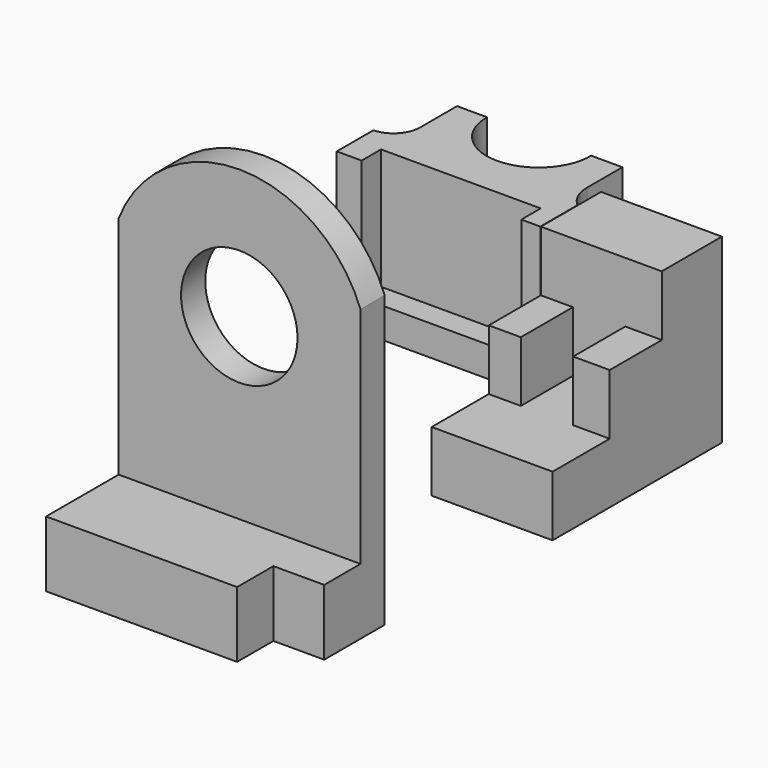
from build123d import *
from build123d import SkipClean  # not in build123d's __all__

# Parameters (mm, degrees)
F0_W      = 25.4
F0_H      = 44.45
F1_DEPTH  = 12.7
F2_W      = 25.4
F2_H      = 29.4602914497
F3_DEPTH  = 12.7
F4_W      = 10.9979929402
F4_H      = 13.6651070789
F5_DEPTH  = 12.7
F7_DEPTH  = 12.7
F8_W      = 50.8
F8_H      = 25.4
F9_DEPTH  = 101.6
F11_DEPTH = 25.4
F12_R     = 12.2295787835
F13_DEPTH = 25.4
F14_R     = 12.2295787835
F15_DEPTH = 19.05
F16_W     = 10.6714690655
F16_H     = 9.525
F17_DEPTH = 25.4
F19_DEPTH = 6.35
F21_DEPTH = 25.4
F23_DEPTH = 25.4


with BuildPart() as f1:
    # F0 (on Top) → F1 (new body)
    with BuildSketch(Plane.XY):
        with Locations((12.7, 22.225)):
            Rectangle(F0_W, F0_H)
    extrude(amount=F1_DEPTH)

    # F2 (on face) → F3 (join)
    with BuildSketch(Plane.XY.offset(12.7)):
        with Locations((12.7, 29.7198542751)):
            Rectangle(F2_W, F2_H)
    extrude(amount=F3_DEPTH)

    # F4 (on face) → F5 (cut)
    with BuildSketch(Plane.XY.offset(25.4)):
        with Locations((12.2352666222, 21.8222620897)):
            Rectangle(F4_W, F4_H)
    extrude(amount=-F5_DEPTH, mode=Mode.SUBTRACT)

    # F6 (on face) → F7 (join)
    with BuildSketch(Plane.XY.offset(25.4)):
        Polygon((25.4, 44.45), (0, 44.45), (0, 28.6548156291), (6.736270152, 28.6548156291), (17.7342630923, 28.6548156291), (25.4, 28.6548156291), align=None)
    extrude(amount=F7_DEPTH)

    # F18 (on Top) → F19 (join)
    with BuildSketch(Plane.XY):
        with BuildLine():
            Line((-3.81, 63.023544848), (-53.6545139277, 63.023544848))
            ThreePointArc((-53.6545139277, 63.023544848), (-56.348590764, 61.9076216843), (-57.4645139277, 59.213544848))
            Line((-57.4645139277, 59.213544848), (-57.4645139277, 38.1405837834))
            Line((-57.4645139277, 38.1405837834), (0, 38.1405837834))
            Line((0, 38.1405837834), (0, 59.213544848))
            ThreePointArc((0, 59.213544848), (-1.1159231637, 61.9076216843), (-3.81, 63.023544848))
        make_face()
    extrude(amount=F19_DEPTH)

    # F20 (on face) → F21 (cut)
    with BuildSketch(Plane.XY.offset(6.35)):
        with BuildLine():
            Line((-16.9094149023, 63.023544848), (-38.7679263949, 63.023544848))
            ThreePointArc((-38.7679263949, 63.023544848), (-27.8386706486, 51.9472434828), (-16.9094149023, 63.023544848))
        make_face()
    extrude(amount=-F21_DEPTH, mode=Mode.SUBTRACT)

    # F22 (on face) → F23 (join)
    with BuildSketch(Plane.XY.offset(6.35)):
        with BuildLine():
            Line((-45.2292449772, 38.1405837834), (-45.2292449772, 43.2271584868))
            Line((-45.2292449772, 43.2271584868), (-11.6853676736, 43.2271584868))
            Line((-11.6853676736, 43.2271584868), (-11.6853676736, 38.1405837834))
            Line((-11.6853676736, 38.1405837834), (-7.6985950582, 38.1405837834))
            Line((-7.6985950582, 38.1405837834), (-7.6985950582, 47.9013063014))
            ThreePointArc((-7.6985950582, 47.9013063014), (-9.6624188313, 50.4964154712), (-10.3597074512, 53.6752492189))
            Line((-10.3597074512, 53.6752492189), (-10.3597074512, 63.023544848))
            Line((-10.3597074512, 63.023544848), (-16.9094149023, 63.023544848))
            ThreePointArc((-16.9094149023, 63.023544848), (-27.8386706486, 51.9472434828), (-38.7679263949, 63.023544848))
            Line((-38.7679263949, 63.023544848), (-45.0917705894, 63.023544848))
            Line((-45.0917705894, 63.023544848), (-45.0917705894, 53.2628260553))
            ThreePointArc((-45.0917705894, 53.2628260553), (-46.6539859613, 49.4227442996), (-50.4532940686, 47.7638281882))
            Line((-50.4532940686, 47.7638281882), (-50.4532940686, 38.1405837834))
            Line((-50.4532940686, 38.1405837834), (-45.2292449772, 38.1405837834))
        make_face()
    with SkipClean():  # cleaning this boolean's faces spoils the solid; the shape is the same uncleaned
        extrude(amount=F23_DEPTH)


with BuildPart() as f9:
    # F8 (on Top) → F9 (new body)
    with BuildSketch(Plane.XY):
        with Locations((-2.7682126224, -53.3297498107)):
            Rectangle(F8_W, F8_H)
    extrude(amount=F9_DEPTH)

    # F10 (on face) → F11 (cut)
    with BuildSketch(Plane.XZ.offset(66.0297498107)):
        with BuildLine():
            ThreePointArc((-28.1682126224, 61.2272843719), (-2.6642465557, 78.5167686352), (22.6317873776, 60.9244629741))
            Line((22.6317873776, 60.9244629741), (22.6317873776, 101.6))
            Line((22.6317873776, 101.6), (-28.1682126224, 101.6))
            Line((-28.1682126224, 101.6), (-28.1682126224, 61.2272843719))
        make_face()
    extrude(amount=-F11_DEPTH, mode=Mode.SUBTRACT)

    # F12 (on face) → F13 (cut)
    with BuildSketch(Plane.XZ.offset(66.0297498107)):
        with Locations((-2.826482869, 51.3007106537)):
            Circle(F12_R)
    extrude(amount=-F13_DEPTH, mode=Mode.SUBTRACT)

    # F14 (on face) → F15 (cut)
    with BuildSketch(Plane.XZ.offset(66.0297498107)):
        with BuildLine():
            Line((-28.1682126224, 61.2272843719), (-28.1682126224, 13.8355828822))
            Line((-28.1682126224, 13.8355828822), (22.6317873776, 13.8355828822))
            Line((22.6317873776, 13.8355828822), (22.6317873776, 60.9244629741))
            ThreePointArc((22.6317873776, 60.9244629741), (-2.6642465557, 78.5167686352), (-28.1682126224, 61.2272843719))
        make_face()
        with Locations((-2.826482869, 51.3007106537)):
            Circle(F14_R, mode=Mode.SUBTRACT)
    extrude(amount=-F15_DEPTH, mode=Mode.SUBTRACT)

    # F16 (on face) → F17 (cut)
    with BuildSketch(Plane.XY.offset(13.8355828822)):
        with Locations((17.2960528448, -61.2672498107)):
            Rectangle(F16_W, F16_H)
    extrude(amount=-F17_DEPTH, mode=Mode.SUBTRACT)


solid = Compound([f1.part, f9.part])
